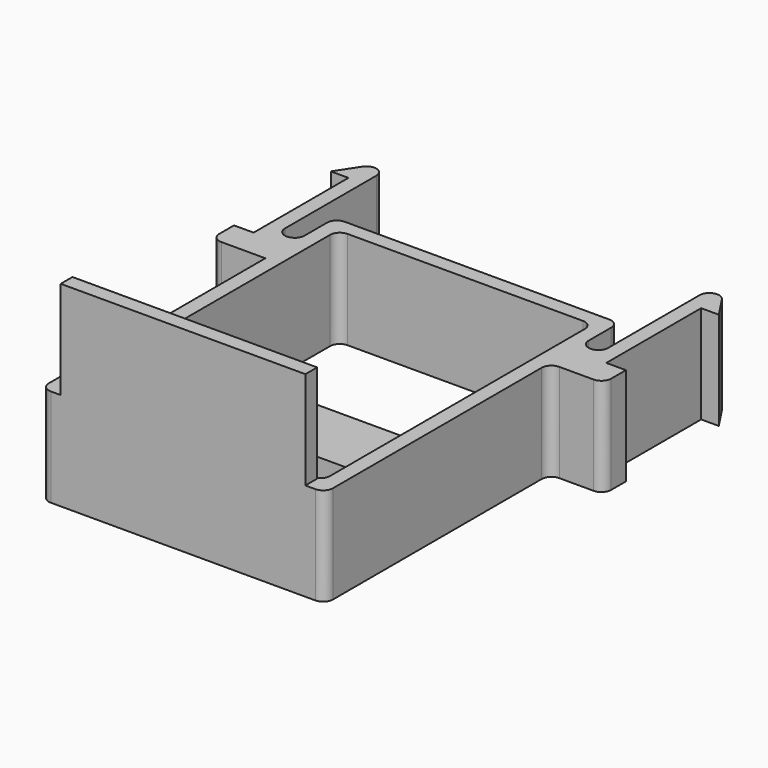
from build123d import *

# Parameters (mm, degrees)
F0_W     = 2
F0_H     = 4
F0_H_2   = 2.8740456328
F1_DEPTH = 10
F2_R     = 0.99999
F0_W_2   = 26
F0_H_3   = 7
F3_DEPTH = 2
F4_W     = 24.9721305105
F4_H     = 10
F5_DEPTH = 1.5


# Not quite as in the source:
# - a fillet or chamfer is up to 0.001 mm smaller than in the source, because OpenCascade refuses the exact size


with BuildPart() as f1:
    # F0 (on Top) → F1 (new body)
    with BuildSketch(Plane.XY):
        Polygon((14.5, 18.75), (-14.5, 18.75), (-14.5, 13.8759543672), (-14.5, 9.8759543672), (-14.5, -18.75), (14.5, -18.75), (14.5, 9.8759543672), (14.5, 13.8759543672), align=None)
        Polygon((-13, 4.7144976147), (-13, 17.25), (13, 17.25), (13, 4.7144976147), (13, -2.2855023853), (13, -17.25), (-13, -17.25), (-13, -2.2855023853), align=None, mode=Mode.SUBTRACT)
        with Locations((-15.5, 11.8759543672)):
            Rectangle(F0_W, F0_H)
        Polygon((-16.5, 9.8759543672), (-16.5, 13.8759543672), (-16.5, 29.8609879265), (-19.8, 24.85), (-18, 24.85), (-18, 12.75), (-18, 9.8759543672), align=None)
        with Locations((15.5, 11.8759543672)):
            Rectangle(F0_W, F0_H)
        Polygon((16.5, 29.8609879265), (16.5, 13.8759543672), (16.5, 9.8759543672), (18, 9.8759543672), (18, 12.75), (18, 24.85), (19.8, 24.85), align=None)
        with Locations((-19, 11.3129771836)):
            Rectangle(F0_W, F0_H_2)
        with Locations((19, 11.3129771836)):
            Rectangle(F0_W, F0_H_2)
    extrude(amount=F1_DEPTH)

    # F2 (radius 1 in the source; OpenCascade refuses exactly that, so slightly less here)
    f2_edges = [f1.edges().sort_by_distance(p)[0] for p in [
        (-14.5, 18.75, 5),
        (-20, 9.875954, 5),
        (14.5, 18.75, 5),
        (20, 9.875954, 5),
        (-13, 17.25, 5),
        (14.5, 9.875954, 5),
        (14.5, -18.75, 5),
        (-14.5, -18.75, 5),
        (-13, -17.25, 5),
        (13, 17.25, 5),
        (13, -17.25, 5),
        (-14.5, 13.875954, 5),
        (16.5, 13.875954, 5),
        (-16.5, 13.875954, 5),
        (14.5, 13.875954, 5),
        (-16.5, 29.860988, 5),
        (16.5, 29.860988, 5),
    ]]
    fillet(f2_edges, radius=F2_R)

    # F0 (on Top) → F3 (join)
    with BuildSketch(Plane.XY):
        with Locations((0, 1.2144976147)):
            Rectangle(F0_W_2, F0_H_3)
    extrude(amount=F3_DEPTH)

    # F4 (on face) → F5 (join)
    with BuildSketch(Plane.XZ.offset(18.75)):
        with Locations((0, 15)):
            Rectangle(F4_W, F4_H)
    extrude(amount=-F5_DEPTH)


solid = f1.part
